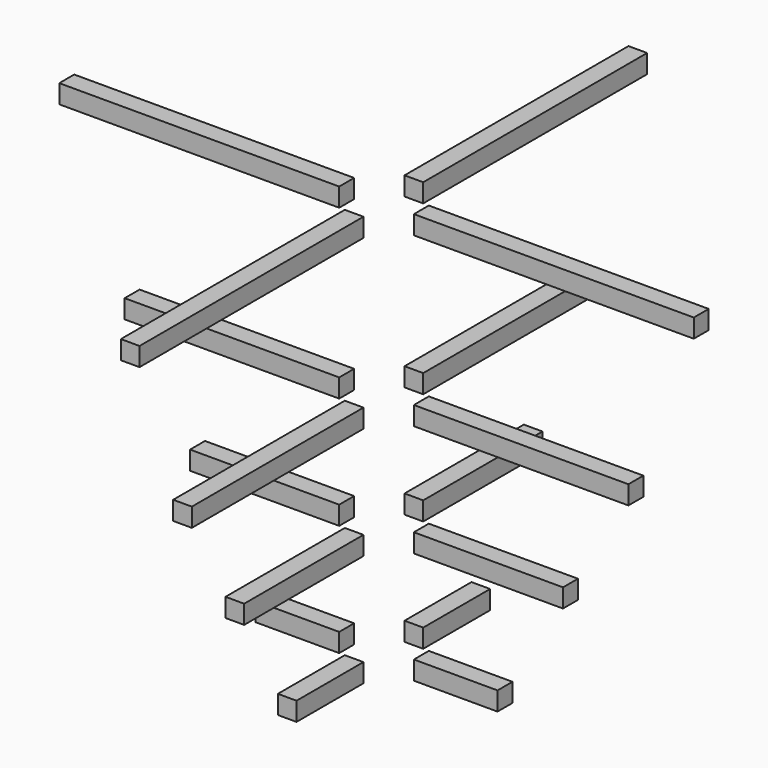
from build123d import *

# Parameters (mm, degrees)
F16_W     = 149.9264546797
F16_H     = 10
F17_DEPTH = 10
F16_W_2   = 10
F16_H_2   = 149.9264546797
F18_W     = 114.9073756323
F18_H     = 10
F19_DEPTH = 10
F18_W_2   = 10
F18_H_2   = 114.9073756323
F20_W     = 79.8749217772
F20_H     = 10
F21_DEPTH = 10
F20_W_2   = 10
F20_H_2   = 79.8749217772
F22_W     = 44.8074069841
F22_H     = 10
F23_DEPTH = 10
F22_W_2   = 10
F22_H_2   = 44.8074069841


# Not quite as in the source:
# - the program builds the solid bodies; features that only make, move or delete a surface that nothing else refers to are left out


with BuildPart() as f17:
    # F16 (on Top) → F17 (new body)
    with BuildSketch(Plane.XY):
        with Locations((-94.9632273398, 0)):
            Rectangle(F16_W, F16_H)
    extrude(amount=-F17_DEPTH)


with BuildPart() as f17b:
    # F16 (on Top) → F17, piece 2 (new body)
    with BuildSketch(Plane.XY):
        with Locations((94.9632273398, 0)):
            Rectangle(F16_W, F16_H)
    extrude(amount=-F17_DEPTH)


with BuildPart() as f17c:
    # F16 (on Top) → F17, piece 3 (new body)
    with BuildSketch(Plane.XY):
        with Locations((0, 94.9632273398)):
            Rectangle(F16_W_2, F16_H_2)
    extrude(amount=-F17_DEPTH)


with BuildPart() as f17d:
    # F16 (on Top) → F17, piece 4 (new body)
    with BuildSketch(Plane.XY):
        with Locations((0, -94.9632273398)):
            Rectangle(F16_W_2, F16_H_2)
    extrude(amount=-F17_DEPTH)


with BuildPart() as f19:
    # F18 (on offset) → F19 (new body)
    with BuildSketch(Plane.XY.offset(-90)):
        with Locations((-77.4536878162, 0)):
            Rectangle(F18_W, F18_H)
    extrude(amount=-F19_DEPTH)


with BuildPart() as f19b:
    # F18 (on offset) → F19, piece 2 (new body)
    with BuildSketch(Plane.XY.offset(-90)):
        with Locations((77.4536878162, 0)):
            Rectangle(F18_W, F18_H)
    extrude(amount=-F19_DEPTH)


with BuildPart() as f19c:
    # F18 (on offset) → F19, piece 3 (new body)
    with BuildSketch(Plane.XY.offset(-90)):
        with Locations((0, -77.4536878162)):
            Rectangle(F18_W_2, F18_H_2)
    extrude(amount=-F19_DEPTH)


with BuildPart() as f19d:
    # F18 (on offset) → F19, piece 4 (new body)
    with BuildSketch(Plane.XY.offset(-90)):
        with Locations((0, 77.4536878162)):
            Rectangle(F18_W_2, F18_H_2)
    extrude(amount=-F19_DEPTH)


with BuildPart() as f21:
    # F20 (on offset) → F21 (new body)
    with BuildSketch(Plane.XY.offset(-150)):
        with Locations((-59.9374608886, 0)):
            Rectangle(F20_W, F20_H)
    extrude(amount=-F21_DEPTH)


with BuildPart() as f21b:
    # F20 (on offset) → F21, piece 2 (new body)
    with BuildSketch(Plane.XY.offset(-150)):
        with Locations((0, 59.9374608886)):
            Rectangle(F20_W_2, F20_H_2)
    extrude(amount=-F21_DEPTH)


with BuildPart() as f21c:
    # F20 (on offset) → F21, piece 3 (new body)
    with BuildSketch(Plane.XY.offset(-150)):
        with Locations((59.9374608886, 0)):
            Rectangle(F20_W, F20_H)
    extrude(amount=-F21_DEPTH)


with BuildPart() as f21d:
    # F20 (on offset) → F21, piece 4 (new body)
    with BuildSketch(Plane.XY.offset(-150)):
        with Locations((0, -59.9374608886)):
            Rectangle(F20_W_2, F20_H_2)
    extrude(amount=-F21_DEPTH)


with BuildPart() as f23:
    # F22 (on offset) → F23 (new body)
    with BuildSketch(Plane.XY.offset(-210)):
        with Locations((-42.403703492, 0)):
            Rectangle(F22_W, F22_H)
    extrude(amount=-F23_DEPTH)


with BuildPart() as f23b:
    # F22 (on offset) → F23, piece 2 (new body)
    with BuildSketch(Plane.XY.offset(-210)):
        with Locations((0, -42.403703492)):
            Rectangle(F22_W_2, F22_H_2)
    extrude(amount=-F23_DEPTH)


with BuildPart() as f23c:
    # F22 (on offset) → F23, piece 3 (new body)
    with BuildSketch(Plane.XY.offset(-210)):
        with Locations((42.403703492, 0)):
            Rectangle(F22_W, F22_H)
    extrude(amount=-F23_DEPTH)


with BuildPart() as f23d:
    # F22 (on offset) → F23, piece 4 (new body)
    with BuildSketch(Plane.XY.offset(-210)):
        with Locations((0, 42.403703492)):
            Rectangle(F22_W_2, F22_H_2)
    extrude(amount=-F23_DEPTH)


solid = Compound([f17.part, f17b.part, f17c.part, f17d.part, f19.part, f19b.part, f19c.part, f19d.part, f21.part, f21b.part, f21c.part, f21d.part, f23.part, f23b.part, f23c.part, f23d.part])
